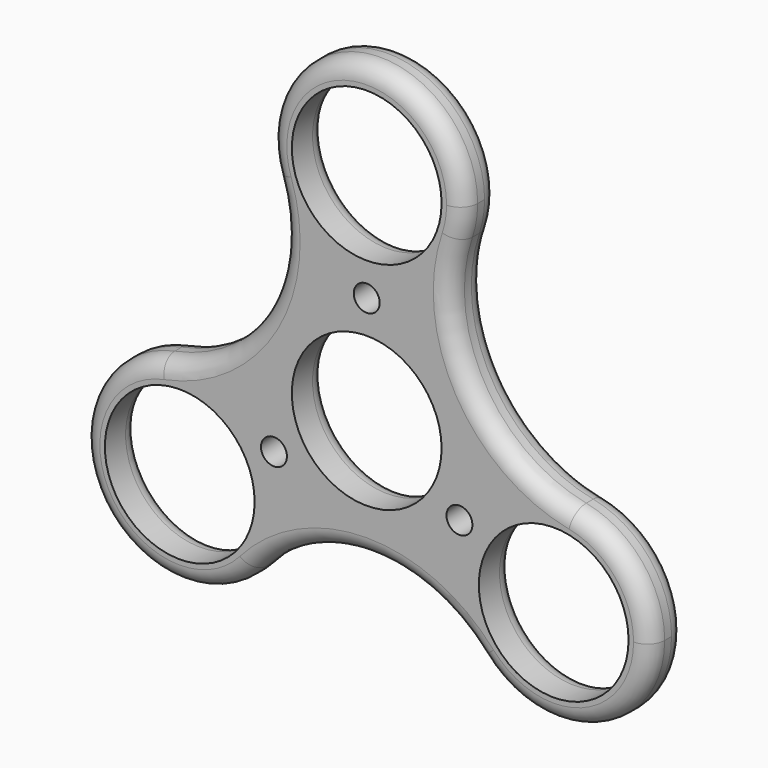
from build123d import *

# Parameters (mm, degrees)
F0_R         = 14.2875
F0_R_2       = 11.0109
F1_DEPTH     = 6.35
F2_R         = 2.54
F3_T2_ANGLE  = 97.7132585674
F3_T4_ANGLE  = 217.7132585674
F3_T6_ANGLE  = 97.7132585674
F3_T8_ANGLE  = 217.7132585674
F3_T10_ANGLE = 97.7132585674
F3_T12_ANGLE = 217.7132585674
F4_R         = 1.905
F5_DEPTH     = 25.4


# Not quite as in the source:
# - a fillet or chamfer that OpenCascade refuses, or shapes differently, is made with other operations: its cross-section is extruded or revolved along the edge and cut away or added


with BuildPart() as f1:
    # F0 (on Front) → F1 (new body)
    with BuildSketch(Plane.XZ):
        with BuildLine():
            ThreePointArc((13.5206938879, 27.1322632123), (0, 17.4625), (-13.5206938879, 27.1322632123))
            ThreePointArc((-13.5206938879, 27.1322632123), (-15.305469781, 8.8366170981), (-30.257576148, -1.8568672225))
            ThreePointArc((-30.257576148, -1.8568672225), (-18.4221394691, -4.8390520266), (-13.2088065702, -15.875))
            ThreePointArc((-13.2088065702, -15.875), (-14.1198733557, -20.8953277493), (-16.7368822601, -25.2753959899))
            ThreePointArc((-16.7368822601, -25.2753959899), (0, -17.6732341963), (16.7368822601, -25.2753959899))
            ThreePointArc((16.7368822601, -25.2753959899), (15.1229686136, -8.73125), (30.257576148, -1.8568672225))
            ThreePointArc((30.257576148, -1.8568672225), (15.305469781, 8.8366170981), (13.5206938879, 27.1322632123))
        make_face()
        Circle(F0_R, mode=Mode.SUBTRACT)
        with BuildLine():
            ThreePointArc((-13.2088065702, -15.875), (-18.4221394691, -4.8390520266), (-30.257576148, -1.8568672225))
            ThreePointArc((-30.257576148, -1.8568672225), (-39.8696445267, -23.01875), (-16.7368822601, -25.2753959899))
            ThreePointArc((-16.7368822601, -25.2753959899), (-14.1198733557, -20.8953277493), (-13.2088065702, -15.875))
        make_face()
        with Locations((-27.4963065702, -15.875)):
            Circle(F0_R_2, mode=Mode.SUBTRACT)
        Circle(F0_R)
        Circle(F0_R_2, mode=Mode.SUBTRACT)
        with BuildLine():
            ThreePointArc((41.7838065702, -15.875), (38.5322545436, -6.8008328989), (30.257576148, -1.8568672225))
            ThreePointArc((30.257576148, -1.8568672225), (15.1229686136, -8.73125), (16.7368822601, -25.2753959899))
            ThreePointArc((16.7368822601, -25.2753959899), (32.5166343194, -29.2514332144), (41.7838065702, -15.875))
        make_face()
        with Locations((27.4963065702, -15.875)):
            Circle(F0_R_2, mode=Mode.SUBTRACT)
        with BuildLine():
            ThreePointArc((13.5206938879, 27.1322632123), (14.0944948503, 29.409514759), (14.2875, 31.75))
            ThreePointArc((14.2875, 31.75), (-2.340485241, 45.8444948503), (-13.5206938879, 27.1322632123))
            ThreePointArc((-13.5206938879, 27.1322632123), (0, 17.4625), (13.5206938879, 27.1322632123))
        make_face()
        with Locations((0, 31.75)):
            Circle(F0_R_2, mode=Mode.SUBTRACT)
    extrude(amount=F1_DEPTH)

    # F2
    f2_edges = [f1.edges().sort_by_distance(p)[0] for p in [
        (-15.30547, -6.35, 8.836617),
    ]]
    fillet(f2_edges, radius=F2_R)

    # F3: fillet of radius 2.54 on 10 edges, made by hand

    # F3_s1 → F3_t2 (revolve, cut)
    with BuildSketch(Plane(origin=(29.4795189524, 0, -5.8068289225), x_dir=(0, 1, 0), z_dir=(0.9811466511, 0, -0.1932647124))):
        with BuildLine():
            ThreePointArc((-2.54, 4.025862694), (-0.7439487758, 3.2819139183), (0, 1.485862694))
            Line((0, 1.485862694), (0, 4.025862694))
            Line((0, 4.025862694), (-2.54, 4.025862694))
        make_face()
    revolve(axis=Axis((34.5528843801, 0, 19.9491170981), (0, 1, 0)), revolution_arc=F3_T2_ANGLE, mode=Mode.SUBTRACT)

    # F3_s3 → F3_t4 (revolve, cut)
    with BuildSketch(Plane(origin=(9.7108981139, 0, 28.4334267654), x_dir=(0, 1, 0), z_dir=(-0.323201175, 0, -0.9463302809))):
        with BuildLine():
            ThreePointArc((0, 1.485862694), (-0.7439487758, 3.2819139183), (-2.54, 4.025862694))
            Line((-2.54, 4.025862694), (0, 4.025862694))
            Line((0, 4.025862694), (0, 1.485862694))
        make_face()
    revolve(axis=Axis((0, 0, 31.75), (0, -1, 0)), revolution_arc=F3_T4_ANGLE, mode=Mode.SUBTRACT)

    # F3_s5 → F3_t6 (revolve, cut)
    with BuildSketch(Plane(origin=(-9.7108981139, 0, 28.4334267654), x_dir=(0, 1, 0), z_dir=(-0.323201175, 0, 0.9463302809))):
        with BuildLine():
            ThreePointArc((0, 1.485862694), (-0.7439487758, 3.2819139183), (-2.54, 4.025862694))
            Line((-2.54, 4.025862694), (0, 4.025862694))
            Line((0, 4.025862694), (0, 1.485862694))
        make_face()
    revolve(axis=Axis((-34.5528843801, 0, 19.9491170981), (0, 1, 0)), revolution_arc=F3_T6_ANGLE, mode=Mode.SUBTRACT)

    # F3_s7 → F3_t8 (revolve, cut)
    with BuildSketch(Plane(origin=(-29.4795189524, 0, -5.8068289225), x_dir=(0, 1, 0), z_dir=(0.9811466511, 0, 0.1932647124))):
        with BuildLine():
            ThreePointArc((0, 1.485862694), (-0.7439487758, 3.2819139183), (-2.54, 4.025862694))
            Line((-2.54, 4.025862694), (0, 4.025862694))
            Line((0, 4.025862694), (0, 1.485862694))
        make_face()
    revolve(axis=Axis((-27.4963065702, 0, -15.875), (0, -1, 0)), revolution_arc=F3_T8_ANGLE, mode=Mode.SUBTRACT)

    # F3_s9 → F3_t10 (revolve, cut)
    with BuildSketch(Plane(origin=(-19.7686208385, 0, -22.6265978429), x_dir=(0, 1, 0), z_dir=(-0.6579454761, 0, -0.7530655685))):
        with BuildLine():
            ThreePointArc((0, 1.485862694), (-0.7439487758, 3.2819139183), (-2.54, 4.025862694))
            Line((-2.54, 4.025862694), (0, 4.025862694))
            Line((0, 4.025862694), (0, 1.485862694))
        make_face()
    revolve(axis=Axis((0, 0, -39.8982341963), (0, 1, 0)), revolution_arc=F3_T10_ANGLE, mode=Mode.SUBTRACT)

    # F3_s11 → F3_t12 (revolve, cut)
    with BuildSketch(Plane(origin=(19.7686208385, 0, -22.6265978429), x_dir=(0, 1, 0), z_dir=(-0.6579454761, 0, 0.7530655685))):
        with BuildLine():
            ThreePointArc((-2.54, 4.025862694), (-0.7439487758, 3.2819139183), (0, 1.485862694))
            Line((0, 1.485862694), (0, 4.025862694))
            Line((0, 4.025862694), (-2.54, 4.025862694))
        make_face()
    revolve(axis=Axis((27.4963065702, 0, -15.875), (0, -1, 0)), revolution_arc=F3_T12_ANGLE, mode=Mode.SUBTRACT)

    # F3_s13 → F3_t14 (revolve, cut)
    with BuildSketch(Plane.XY.offset(-15.875)):
        with BuildLine():
            ThreePointArc((-13.9454065702, 0), (-15.7414577944, -0.7439487758), (-16.4854065702, -2.54))
            Line((-16.4854065702, -2.54), (-16.4854065702, 0))
            Line((-16.4854065702, 0), (-13.9454065702, 0))
        make_face()
    revolve(axis=Axis((-27.4963065702, 0, -15.875), (0, -1, 0)), mode=Mode.SUBTRACT)

    # F3_s15 → F3_t16 (revolve, cut)
    with BuildSketch(Plane.XY):
        with BuildLine():
            ThreePointArc((13.5509, 0), (11.7548487758, -0.7439487758), (11.0109, -2.54))
            Line((11.0109, -2.54), (11.0109, 0))
            Line((11.0109, 0), (13.5509, 0))
        make_face()
    revolve(axis=Axis((0, 0, 0), (0, -1, 0)), mode=Mode.SUBTRACT)

    # F3_s17 → F3_t18 (revolve, cut)
    with BuildSketch(Plane.XY.offset(-15.875)):
        with BuildLine():
            ThreePointArc((41.0472065702, 0), (39.2511553459, -0.7439487758), (38.5072065702, -2.54))
            Line((38.5072065702, -2.54), (38.5072065702, 0))
            Line((38.5072065702, 0), (41.0472065702, 0))
        make_face()
    revolve(axis=Axis((27.4963065702, 0, -15.875), (0, -1, 0)), mode=Mode.SUBTRACT)

    # F3_s19 → F3_t20 (revolve, cut)
    with BuildSketch(Plane.XY.offset(31.75)):
        with BuildLine():
            ThreePointArc((13.5509, 0), (11.7548487758, -0.7439487758), (11.0109, -2.54))
            Line((11.0109, -2.54), (11.0109, 0))
            Line((11.0109, 0), (13.5509, 0))
        make_face()
    revolve(axis=Axis((0, 0, 31.75), (0, -1, 0)), mode=Mode.SUBTRACT)

    # F4 (on face) → F5 (cut)
    with BuildSketch(Plane.XZ.offset(6.35)):
        with Locations((-13.6389745453, -8.4374256665)):
            Circle(F4_R)
        with Locations((13.6389745453, -8.4374256665)):
            Circle(F4_R)
        with Locations((0, 15.875)):
            Circle(F4_R)
    extrude(amount=-F5_DEPTH, mode=Mode.SUBTRACT)


solid = f1.part
